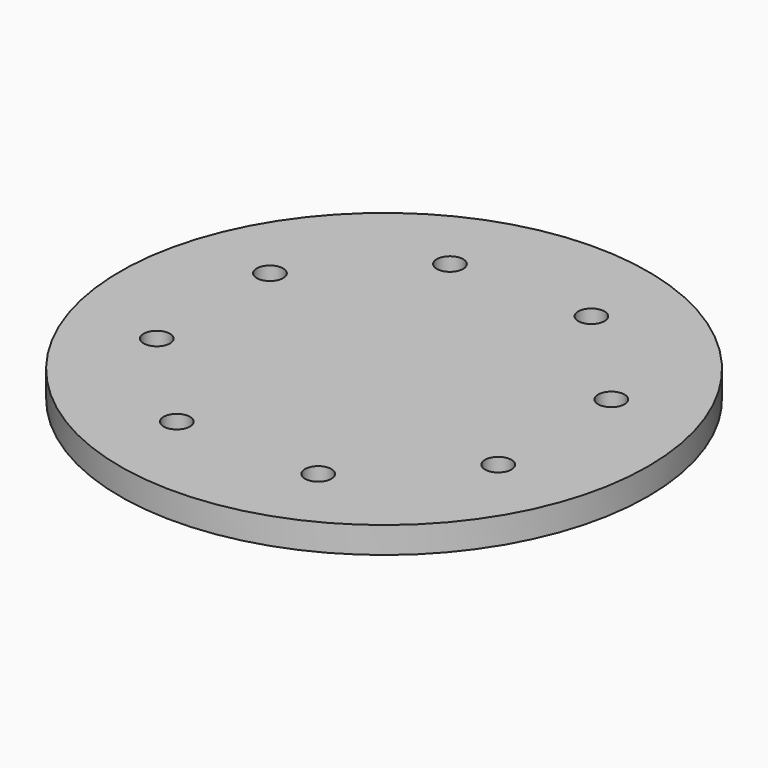
from build123d import *

# Parameters (mm, degrees)
F0_R     = 200
F0_R_2   = 10
F1_DEPTH = 20


# Not quite as in the source:
# - a feature names something its author has since deleted; it is built from what else it names


with BuildPart() as f1:
    # F0 (on Top) → F1 (new body)
    with BuildSketch(Plane.XY):
        Circle(F0_R)
        with Locations((-53.5756805311, -129.3431345516)):
            Circle(F0_R_2, mode=Mode.SUBTRACT)
        with Locations((-129.3431345516, -53.5756805311)):
            Circle(F0_R_2, mode=Mode.SUBTRACT)
        with Locations((53.5756805311, -129.3431345516)):
            Circle(F0_R_2, mode=Mode.SUBTRACT)
        with Locations((129.3431345516, -53.5756805311)):
            Circle(F0_R_2, mode=Mode.SUBTRACT)
        with Locations((-129.3431345516, 53.5756805311)):
            Circle(F0_R_2, mode=Mode.SUBTRACT)
        with Locations((-53.5756805311, 129.3431345516)):
            Circle(F0_R_2, mode=Mode.SUBTRACT)
        with Locations((129.3431345516, 53.5756805311)):
            Circle(F0_R_2, mode=Mode.SUBTRACT)
        with BuildLine():
            ThreePointArc((49.7488462075, 120.1043392265), (48.0199782009, 137.6578306746), (63.5756805311, 129.3431345516))
            ThreePointArc((63.5756805311, 129.3431345516), (59.1313828613, 121.0284384286), (49.7488462075, 120.1043392265))
        make_face(mode=Mode.SUBTRACT)
    extrude(amount=F1_DEPTH)


solid = f1.part
